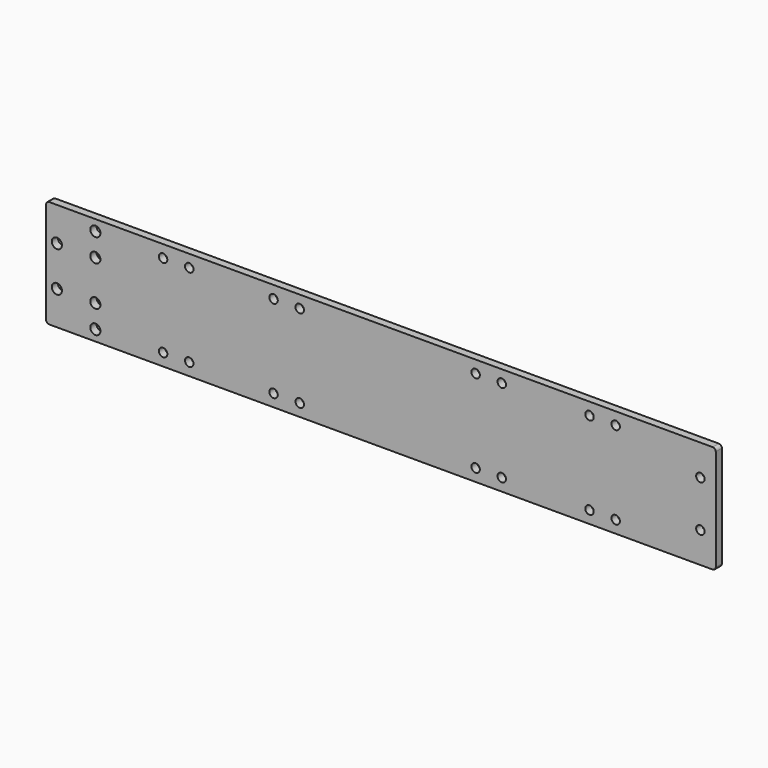
from build123d import *

# Parameters (mm, degrees)
F0_W     = 435
F0_H     = 70
F1_DEPTH = 5
F2_R     = 2
F4_D     = 6.6
F6_D     = 5.5
F8_D     = 5.5
F10_D    = 5.5


# Not quite as in the source:
# - a feature names something its author has since deleted; it is built from what else it names


with BuildPart() as f1:
    # F0 (on Front) → F1 (new body)
    with BuildSketch(Plane.XZ):
        Rectangle(F0_W, F0_H)
    extrude(amount=F1_DEPTH)

    # F2
    f2_edges = [f1.edges().sort_by_distance(p)[0] for p in [
        (217.5, -2.5, 35),
        (217.5, -2.5, -35),
        (-217.5, -2.5, 35),
        (-217.5, -2.5, -35),
    ]]
    fillet(f2_edges, radius=F2_R)

    # F4 (through all)
    with Locations(Plane.XZ.offset(5)):
        with Locations((-185.5, 13), (-210.5, 13), (-210.5, -13), (-185.5, -13), (-185.5, 28), (-185.5, -28)):
            Hole(F4_D / 2)

    # F6 (through all)
    with Locations(Plane.XZ.offset(5)):
        with Locations((-141.5, 27), (-124.5, 27), (-141.5, -27), (-124.5, -27)):
            Hole(F6_D / 2)

    # F8 (through all)
    with Locations(Plane.XZ.offset(5)):
        with Locations((-69.75, 27), (-52.75, 27), (-69.75, -27), (-52.75, -27), (61.5, 27), (78.5, 27), (61.5, -27), (78.5, -27), (135.5, 27), (152.5, 27), (135.5, -27), (152.5, -27)):
            Hole(F8_D / 2)

    # F10 (through all)
    with Locations(Plane.XZ.offset(5)):
        with Locations((207.5, 15), (207.5, -15)):
            Hole(F10_D / 2)


solid = f1.part
